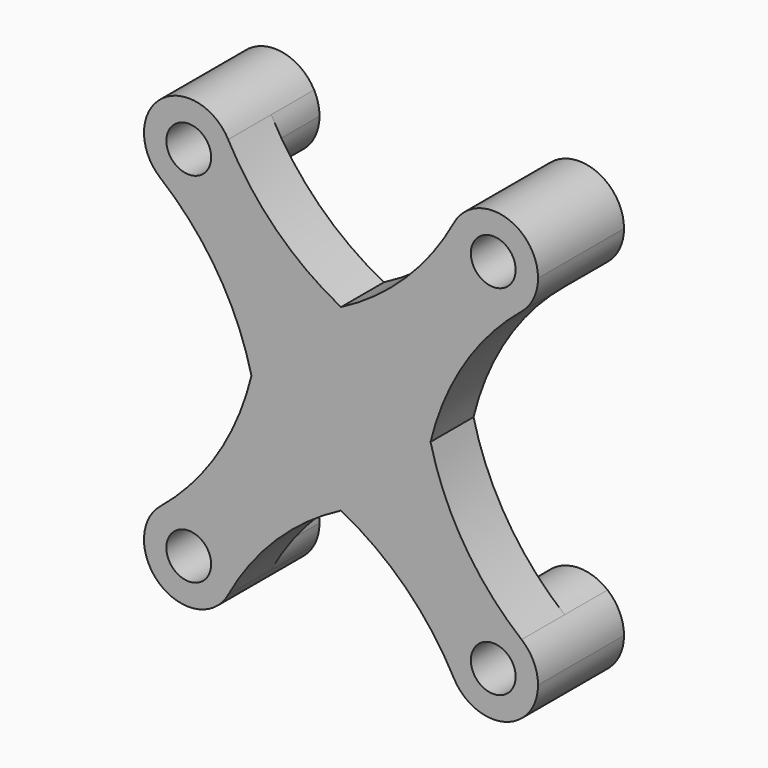
from build123d import *

# Parameters (mm, degrees)
F0_R     = 2.5
F1_DEPTH = 12
F2_START = 6
F2_DEPTH = 6


# Not quite as in the source:
# - a feature names something its author has since deleted; it is built from what else it names


with BuildPart() as f1:
    # F0 (on Front) → F1 (new body)
    with BuildSketch(Plane.XZ):
        with BuildLine():
            ThreePointArc((-20.1639063661, 16.1283470576), (-14.8575168414, 15.4822831081), (-12, 20))
            ThreePointArc((-12, 20), (-12.1526927453, 21.2262187321), (-12.6014449516, 22.3775435823))
            ThreePointArc((-12.6014449516, 22.3775435823), (-20.1849966473, 23.8543217765), (-20.1639063661, 16.1283470576))
        make_face()
        with Locations((-17, 20)):
            Circle(F0_R, mode=Mode.SUBTRACT)
    extrude(amount=F1_DEPTH)



with BuildPart() as f1b:
    # F0 (on Front) → F1, piece 2 (new body)
    with BuildSketch(Plane.XZ):
        with BuildLine():
            ThreePointArc((22, 20), (18.2262187321, 24.8473072547), (12.6014449516, 22.3775435823))
            ThreePointArc((12.6014449516, 22.3775435823), (13.8150033527, 16.1456782235), (20.1639063661, 16.1283470576))
            ThreePointArc((20.1639063661, 16.1283470576), (21.5177168919, 17.8575168414), (22, 20))
        make_face()
        with Locations((17, 20)):
            Circle(F0_R, mode=Mode.SUBTRACT)
    extrude(amount=F1_DEPTH)


with BuildPart() as f1c:
    # F0 (on Front) → F1, piece 3 (new body)
    with BuildSketch(Plane.XZ):
        with BuildLine():
            ThreePointArc((22, -20), (21.5177168919, -17.8575168414), (20.1639063661, -16.1283470576))
            ThreePointArc((20.1639063661, -16.1283470576), (13.8150033527, -16.1456782235), (12.6014449516, -22.3775435823))
            ThreePointArc((12.6014449516, -22.3775435823), (18.2262187321, -24.8473072547), (22, -20))
        make_face()
        with Locations((17, -20)):
            Circle(F0_R, mode=Mode.SUBTRACT)
    extrude(amount=F1_DEPTH)


with BuildPart() as f1d:
    # F0 (on Front) → F1, piece 4 (new body)
    with BuildSketch(Plane.XZ):
        with BuildLine():
            ThreePointArc((-12, -20), (-14.8575168414, -15.4822831081), (-20.1639063661, -16.1283470576))
            ThreePointArc((-20.1639063661, -16.1283470576), (-20.1849966473, -23.8543217765), (-12.6014449516, -22.3775435823))
            ThreePointArc((-12.6014449516, -22.3775435823), (-12.1526927453, -21.2262187321), (-12, -20))
        make_face()
        with Locations((-17, -20)):
            Circle(F0_R, mode=Mode.SUBTRACT)
    extrude(amount=F1_DEPTH)


with BuildPart() as f1_1:
    add(f1.part)

    add(f1b.part)  # F2 merges F1b

    add(f1c.part)  # F2 merges F1c

    add(f1d.part)  # F2 merges F1d
    # F0 (on Front) → F2 (join)
    with BuildSketch(Plane.XZ.offset(F2_START)):
        with BuildLine():
            ThreePointArc((-12.6014449516, 22.3775435823), (-12.1526927453, 21.2262187321), (-12, 20))
            ThreePointArc((-12, 20), (-14.8575168414, 15.4822831081), (-20.1639063661, 16.1283470576))
            ThreePointArc((-20.1639063661, 16.1283470576), (-13.766762281, 8.8929923243), (-10, 0))
            ThreePointArc((-10, 0), (-7.0710678119, 7.0710678119), (0, 10))
            ThreePointArc((0, 10), (-7.2323271671, 15.2403150028), (-12.6014449516, 22.3775435823))
        make_face()
        with BuildLine():
            ThreePointArc((10, 0), (7.0710678119, 7.0710678119), (0, 10))
            ThreePointArc((0, 10), (-7.0710678119, 7.0710678119), (-10, 0))
            ThreePointArc((-10, 0), (-7.0710678119, -7.0710678119), (0, -10))
            ThreePointArc((0, -10), (7.0710678119, -7.0710678119), (10, 0))
        make_face()
        with BuildLine():
            ThreePointArc((0, -10), (-7.0710678119, -7.0710678119), (-10, 0))
            ThreePointArc((-10, 0), (-13.766762281, -8.8929923243), (-20.1639063661, -16.1283470576))
            ThreePointArc((-20.1639063661, -16.1283470576), (-14.8575168414, -15.4822831081), (-12, -20))
            ThreePointArc((-12, -20), (-12.1526927453, -21.2262187321), (-12.6014449516, -22.3775435823))
            ThreePointArc((-12.6014449516, -22.3775435823), (-7.2323271671, -15.2403150028), (0, -10))
        make_face()
        with BuildLine():
            ThreePointArc((20.1639063661, -16.1283470576), (13.766762281, -8.8929923243), (10, 0))
            ThreePointArc((10, 0), (7.0710678119, -7.0710678119), (0, -10))
            ThreePointArc((0, -10), (7.2323271671, -15.2403150028), (12.6014449516, -22.3775435823))
            ThreePointArc((12.6014449516, -22.3775435823), (13.8150033527, -16.1456782235), (20.1639063661, -16.1283470576))
        make_face()
        with BuildLine():
            ThreePointArc((12.6014449516, 22.3775435823), (7.2323271671, 15.2403150028), (0, 10))
            ThreePointArc((0, 10), (7.0710678119, 7.0710678119), (10, 0))
            ThreePointArc((10, 0), (13.766762281, 8.8929923243), (20.1639063661, 16.1283470576))
            ThreePointArc((20.1639063661, 16.1283470576), (13.8150033527, 16.1456782235), (12.6014449516, 22.3775435823))
        make_face()
    extrude(amount=F2_DEPTH)


solid = f1_1.part
